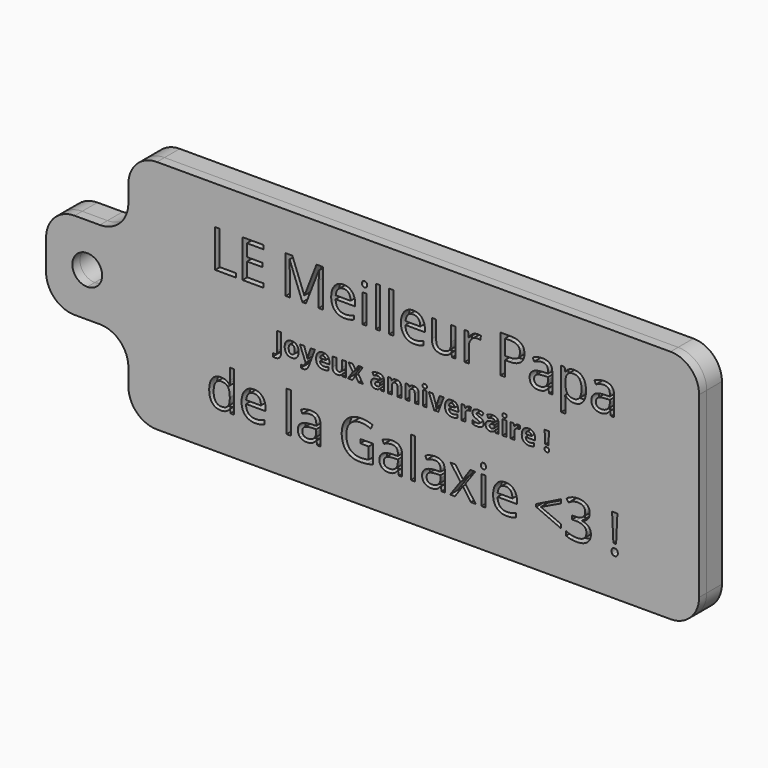
from build123d import *

# Parameters (mm, degrees)
F0_W         = 0.4505208333
F0_H         = 4.2213541667
F0_H_2       = 2.9730902778
F0_W_2       = 8.6528608203
F0_H_3       = 9.189594537
F1_DEPTH     = 1
F2_W         = 8.6528608203
F2_H         = 9.189594537
F3_DEPTH     = 2
F4_R         = 3
F4_2_R       = 3
F6_DEPTH     = 3.001
F7_TEXT_SIZE = 2.7777777778
F8_DEPTH     = 1


# Not quite as in the source:
# - Text() gives the source's letters only with a copy of the font that has no kerning and outlines rounded to 1/6400 em; it was checked with that copy


with BuildPart() as f1:
    # F0 (on Front) → F1 (new body)
    with BuildSketch(Plane.XZ):
        Polygon((-30, -12.3789965568), (30, -12.3789965568), (30, 12.3789965568), (-30, 12.3789965568), (-30, 4.5947972685), (-30, -4.5947972685), align=None)
        with BuildLine():
            Line((-19.2547743056, -8.3789965568), (-19.3146701389, -7.9805590568))
            Line((-19.3146701389, -7.9805590568), (-19.3389756944, -7.9805590568))
            add(Edge.make_bspline(
                [(-19.3389756944, -7.9805590568), (-19.6506076389, -8.4336840568), (-20.2721354167, -8.4336840568)],
                knots=[0, 0, 0, 1, 1, 1], degree=2))
            add(Edge.make_bspline(
                [(-20.2721354167, -8.4336840568), (-20.85546875, -8.4336840568), (-21.1796875, -8.034812529)],
                knots=[0, 0, 0, 1, 1, 1], degree=2))
            add(Edge.make_bspline(
                [(-21.1796875, -8.034812529), (-21.50390625, -7.6359410012), (-21.50390625, -6.9006979457)],
                knots=[0, 0, 0, 1, 1, 1], degree=2))
            add(Edge.make_bspline(
                [(-21.50390625, -6.9006979457), (-21.50390625, -6.1654548901), (-21.1783854167, -5.7583368345)],
                knots=[0, 0, 0, 1, 1, 1], degree=2))
            add(Edge.make_bspline(
                [(-21.1783854167, -5.7583368345), (-20.8528645833, -5.351218779), (-20.2721354167, -5.351218779)],
                knots=[0, 0, 0, 1, 1, 1], degree=2))
            add(Edge.make_bspline(
                [(-20.2721354167, -5.351218779), (-19.6671006944, -5.351218779), (-19.3441840278, -5.7913229457)],
                knots=[0, 0, 0, 1, 1, 1], degree=2))
            Line((-19.3441840278, -5.7913229457), (-19.30859375, -5.7913229457))
            Line((-19.30859375, -5.7913229457), (-19.3276909722, -5.5769132234))
            Line((-19.3276909722, -5.5769132234), (-19.3389756944, -5.3677118345))
            Line((-19.3389756944, -5.3677118345), (-19.3389756944, -4.1576423901))
            Line((-19.3389756944, -4.1576423901), (-18.8884548611, -4.1576423901))
            Line((-18.8884548611, -4.1576423901), (-18.8884548611, -8.3789965568))
            Line((-18.8884548611, -8.3789965568), (-19.2547743056, -8.3789965568))
        make_face(mode=Mode.SUBTRACT)
        with BuildLine():
            add(Edge.make_bspline(
                [(-16.1636284722, -8.3885451679), (-16.3763020833, -8.4336840568), (-16.6775173611, -8.4336840568)],
                knots=[0, 0, 0, 1, 1, 1], degree=2))
            add(Edge.make_bspline(
                [(-16.6775173611, -8.4336840568), (-17.3363715278, -8.4336840568), (-17.7178819444, -8.0317743345)],
                knots=[0, 0, 0, 1, 1, 1], degree=2))
            add(Edge.make_bspline(
                [(-17.7178819444, -8.0317743345), (-18.0993923611, -7.6298646123), (-18.0993923611, -6.9171910012)],
                knots=[0, 0, 0, 1, 1, 1], degree=2))
            add(Edge.make_bspline(
                [(-18.0993923611, -6.9171910012), (-18.0993923611, -6.1975729457), (-17.7452256944, -5.7743958623)],
                knots=[0, 0, 0, 1, 1, 1], degree=2))
            add(Edge.make_bspline(
                [(-17.7452256944, -5.7743958623), (-17.3910590278, -5.351218779), (-16.7938368056, -5.351218779)],
                knots=[0, 0, 0, 1, 1, 1], degree=2))
            add(Edge.make_bspline(
                [(-16.7938368056, -5.351218779), (-16.2356770833, -5.351218779), (-15.91015625, -5.7188403068)],
                knots=[0, 0, 0, 1, 1, 1], degree=2))
            add(Edge.make_bspline(
                [(-15.91015625, -5.7188403068), (-15.5846354167, -6.0864618345), (-15.5846354167, -6.6888923901)],
                knots=[0, 0, 0, 1, 1, 1], degree=2))
            Line((-15.5846354167, -6.6888923901), (-15.5846354167, -6.9736146123))
            Line((-15.5846354167, -6.9736146123), (-17.6323784722, -6.9736146123))
            add(Edge.make_bspline(
                [(-17.6323784722, -6.9736146123), (-17.6184895833, -7.4970521123), (-17.3676215278, -7.7683194734)],
                knots=[0, 0, 0, 1, 1, 1], degree=2))
            add(Edge.make_bspline(
                [(-17.3676215278, -7.7683194734), (-17.1167534722, -8.0395868345), (-16.6610243056, -8.0395868345)],
                knots=[0, 0, 0, 1, 1, 1], degree=2))
            add(Edge.make_bspline(
                [(-16.6610243056, -8.0395868345), (-16.1809895833, -8.0395868345), (-15.7122395833, -7.8390660012)],
                knots=[0, 0, 0, 1, 1, 1], degree=2))
            Line((-15.7122395833, -7.8390660012), (-15.7122395833, -8.2409757234))
            add(Edge.make_bspline(
                [(-15.7122395833, -8.2409757234), (-15.9509548611, -8.343406279), (-16.1636284722, -8.3885451679)],
                knots=[0, 0, 0, 1, 1, 1], degree=2))
        make_face(mode=Mode.SUBTRACT)
        with Locations((-13.1475694444, -6.2683194734)):
            Rectangle(F0_W, F0_H, mode=Mode.SUBTRACT)
        with BuildLine():
            Line((-9.8051215278, -8.3789965568), (-10.1393229167, -8.3789965568))
            Line((-10.1393229167, -8.3789965568), (-10.2287326389, -7.9553854457))
            Line((-10.2287326389, -7.9553854457), (-10.2504340278, -7.9553854457))
            add(Edge.make_bspline(
                [(-10.2504340278, -7.9553854457), (-10.47265625, -8.2348993345), (-10.6935763889, -8.3342916957)],
                knots=[0, 0, 0, 1, 1, 1], degree=2))
            add(Edge.make_bspline(
                [(-10.6935763889, -8.3342916957), (-10.9144965278, -8.4336840568), (-11.24609375, -8.4336840568)],
                knots=[0, 0, 0, 1, 1, 1], degree=2))
            add(Edge.make_bspline(
                [(-11.24609375, -8.4336840568), (-11.6879340278, -8.4336840568), (-11.9388020833, -8.2053854457)],
                knots=[0, 0, 0, 1, 1, 1], degree=2))
            add(Edge.make_bspline(
                [(-11.9388020833, -8.2053854457), (-12.1896701389, -7.9770868345), (-12.1896701389, -7.5569479457)],
                knots=[0, 0, 0, 1, 1, 1], degree=2))
            add(Edge.make_bspline(
                [(-12.1896701389, -7.5569479457), (-12.1896701389, -6.6567743345), (-10.7495659722, -6.6133715568)],
                knots=[0, 0, 0, 1, 1, 1], degree=2))
            Line((-10.7495659722, -6.6133715568), (-10.2452256944, -6.5968785012))
            Line((-10.2452256944, -6.5968785012), (-10.2452256944, -6.4119826679))
            add(Edge.make_bspline(
                [(-10.2452256944, -6.4119826679), (-10.2452256944, -6.062156279), (-10.3953993056, -5.8954896123)],
                knots=[0, 0, 0, 1, 1, 1], degree=2))
            add(Edge.make_bspline(
                [(-10.3953993056, -5.8954896123), (-10.5455729167, -5.7288229457), (-10.8771701389, -5.7288229457)],
                knots=[0, 0, 0, 1, 1, 1], degree=2))
            add(Edge.make_bspline(
                [(-10.8771701389, -5.7288229457), (-11.2486979167, -5.7288229457), (-11.7174479167, -5.9562535012)],
                knots=[0, 0, 0, 1, 1, 1], degree=2))
            Line((-11.7174479167, -5.9562535012), (-11.8563368056, -5.6116354457))
            add(Edge.make_bspline(
                [(-11.8563368056, -5.6116354457), (-11.63671875, -5.4927118345), (-11.375, -5.4250035012)],
                knots=[0, 0, 0, 1, 1, 1], degree=2))
            add(Edge.make_bspline(
                [(-11.375, -5.4250035012), (-11.11328125, -5.3572951679), (-10.8493923611, -5.3572951679)],
                knots=[0, 0, 0, 1, 1, 1], degree=2))
            add(Edge.make_bspline(
                [(-10.8493923611, -5.3572951679), (-10.3181423611, -5.3572951679), (-10.0616319444, -5.5929722512)],
                knots=[0, 0, 0, 1, 1, 1], degree=2))
            add(Edge.make_bspline(
                [(-10.0616319444, -5.5929722512), (-9.8051215278, -5.8286493345), (-9.8051215278, -6.3494826679)],
                knots=[0, 0, 0, 1, 1, 1], degree=2))
            Line((-9.8051215278, -6.3494826679), (-9.8051215278, -8.3789965568))
        make_face(mode=Mode.SUBTRACT)
        with BuildLine():
            Line((-5.6219618056, -6.7131979457), (-5.6219618056, -6.3008715568))
            Line((-5.6219618056, -6.3008715568), (-4.2738715278, -6.3008715568))
            Line((-4.2738715278, -6.3008715568), (-4.2738715278, -8.2296910012))
            add(Edge.make_bspline(
                [(-4.2738715278, -8.2296910012), (-4.5889756944, -8.3303854457), (-4.9144965278, -8.3820347512)],
                knots=[0, 0, 0, 1, 1, 1], degree=2))
            add(Edge.make_bspline(
                [(-4.9144965278, -8.3820347512), (-5.2400173611, -8.4336840568), (-5.6688368056, -8.4336840568)],
                knots=[0, 0, 0, 1, 1, 1], degree=2))
            add(Edge.make_bspline(
                [(-5.6688368056, -8.4336840568), (-6.5690104167, -8.4336840568), (-7.0707465278, -7.8976597512)],
                knots=[0, 0, 0, 1, 1, 1], degree=2))
            add(Edge.make_bspline(
                [(-7.0707465278, -7.8976597512), (-7.5724826389, -7.3616354457), (-7.5724826389, -6.3963576679)],
                knots=[0, 0, 0, 1, 1, 1], degree=2))
            add(Edge.make_bspline(
                [(-7.5724826389, -6.3963576679), (-7.5724826389, -5.7774340568), (-7.32421875, -5.312156279)],
                knots=[0, 0, 0, 1, 1, 1], degree=2))
            add(Edge.make_bspline(
                [(-7.32421875, -5.312156279), (-7.0759548611, -4.8468785012), (-6.609375, -4.6016528068)],
                knots=[0, 0, 0, 1, 1, 1], degree=2))
            add(Edge.make_bspline(
                [(-6.609375, -4.6016528068), (-6.1427951389, -4.3564271123), (-5.5169270833, -4.3564271123)],
                knots=[0, 0, 0, 1, 1, 1], degree=2))
            add(Edge.make_bspline(
                [(-5.5169270833, -4.3564271123), (-4.8815104167, -4.3564271123), (-4.3337673611, -4.5890660012)],
                knots=[0, 0, 0, 1, 1, 1], degree=2))
            Line((-4.3337673611, -4.5890660012), (-4.5125868056, -4.9961840568))
            add(Edge.make_bspline(
                [(-4.5125868056, -4.9961840568), (-5.0499131944, -4.7687535012), (-5.5464409722, -4.7687535012)],
                knots=[0, 0, 0, 1, 1, 1], degree=2))
            add(Edge.make_bspline(
                [(-5.5464409722, -4.7687535012), (-6.2703993056, -4.7687535012), (-6.6775173611, -5.1997430845)],
                knots=[0, 0, 0, 1, 1, 1], degree=2))
            add(Edge.make_bspline(
                [(-6.6775173611, -5.1997430845), (-7.0846354167, -5.6307326679), (-7.0846354167, -6.3963576679)],
                knots=[0, 0, 0, 1, 1, 1], degree=2))
            add(Edge.make_bspline(
                [(-7.0846354167, -6.3963576679), (-7.0846354167, -7.1993090568), (-6.6927083333, -7.6142396123)],
                knots=[0, 0, 0, 1, 1, 1], degree=2))
            add(Edge.make_bspline(
                [(-6.6927083333, -7.6142396123), (-6.30078125, -8.0291701679), (-5.5412326389, -8.0291701679)],
                knots=[0, 0, 0, 1, 1, 1], degree=2))
            add(Edge.make_bspline(
                [(-5.5412326389, -8.0291701679), (-5.12890625, -8.0291701679), (-4.7356770833, -7.9336840568)],
                knots=[0, 0, 0, 1, 1, 1], degree=2))
            Line((-4.7356770833, -7.9336840568), (-4.7356770833, -6.7131979457))
            Line((-4.7356770833, -6.7131979457), (-5.6219618056, -6.7131979457))
        make_face(mode=Mode.SUBTRACT)
        with BuildLine():
            Line((-1.2278645833, -8.3789965568), (-1.5620659722, -8.3789965568))
            Line((-1.5620659722, -8.3789965568), (-1.6514756944, -7.9553854457))
            Line((-1.6514756944, -7.9553854457), (-1.6731770833, -7.9553854457))
            add(Edge.make_bspline(
                [(-1.6731770833, -7.9553854457), (-1.8953993056, -8.2348993345), (-2.1163194444, -8.3342916957)],
                knots=[0, 0, 0, 1, 1, 1], degree=2))
            add(Edge.make_bspline(
                [(-2.1163194444, -8.3342916957), (-2.3372395833, -8.4336840568), (-2.6688368056, -8.4336840568)],
                knots=[0, 0, 0, 1, 1, 1], degree=2))
            add(Edge.make_bspline(
                [(-2.6688368056, -8.4336840568), (-3.1106770833, -8.4336840568), (-3.3615451389, -8.2053854457)],
                knots=[0, 0, 0, 1, 1, 1], degree=2))
            add(Edge.make_bspline(
                [(-3.3615451389, -8.2053854457), (-3.6124131944, -7.9770868345), (-3.6124131944, -7.5569479457)],
                knots=[0, 0, 0, 1, 1, 1], degree=2))
            add(Edge.make_bspline(
                [(-3.6124131944, -7.5569479457), (-3.6124131944, -6.6567743345), (-2.1723090278, -6.6133715568)],
                knots=[0, 0, 0, 1, 1, 1], degree=2))
            Line((-2.1723090278, -6.6133715568), (-1.66796875, -6.5968785012))
            Line((-1.66796875, -6.5968785012), (-1.66796875, -6.4119826679))
            add(Edge.make_bspline(
                [(-1.66796875, -6.4119826679), (-1.66796875, -6.062156279), (-1.8181423611, -5.8954896123)],
                knots=[0, 0, 0, 1, 1, 1], degree=2))
            add(Edge.make_bspline(
                [(-1.8181423611, -5.8954896123), (-1.9683159722, -5.7288229457), (-2.2999131944, -5.7288229457)],
                knots=[0, 0, 0, 1, 1, 1], degree=2))
            add(Edge.make_bspline(
                [(-2.2999131944, -5.7288229457), (-2.6714409722, -5.7288229457), (-3.1401909722, -5.9562535012)],
                knots=[0, 0, 0, 1, 1, 1], degree=2))
            Line((-3.1401909722, -5.9562535012), (-3.2790798611, -5.6116354457))
            add(Edge.make_bspline(
                [(-3.2790798611, -5.6116354457), (-3.0594618056, -5.4927118345), (-2.7977430556, -5.4250035012)],
                knots=[0, 0, 0, 1, 1, 1], degree=2))
            add(Edge.make_bspline(
                [(-2.7977430556, -5.4250035012), (-2.5360243056, -5.3572951679), (-2.2721354167, -5.3572951679)],
                knots=[0, 0, 0, 1, 1, 1], degree=2))
            add(Edge.make_bspline(
                [(-2.2721354167, -5.3572951679), (-1.7408854167, -5.3572951679), (-1.484375, -5.5929722512)],
                knots=[0, 0, 0, 1, 1, 1], degree=2))
            add(Edge.make_bspline(
                [(-1.484375, -5.5929722512), (-1.2278645833, -5.8286493345), (-1.2278645833, -6.3494826679)],
                knots=[0, 0, 0, 1, 1, 1], degree=2))
            Line((-1.2278645833, -6.3494826679), (-1.2278645833, -8.3789965568))
        make_face(mode=Mode.SUBTRACT)
        with Locations((-0.0755208333, -6.2683194734)):
            Rectangle(F0_W, F0_H, mode=Mode.SUBTRACT)
        with BuildLine():
            Line((3.2669270833, -8.3789965568), (2.9327256944, -8.3789965568))
            Line((2.9327256944, -8.3789965568), (2.8433159722, -7.9553854457))
            Line((2.8433159722, -7.9553854457), (2.8216145833, -7.9553854457))
            add(Edge.make_bspline(
                [(2.8216145833, -7.9553854457), (2.5993923611, -8.2348993345), (2.3784722222, -8.3342916957)],
                knots=[0, 0, 0, 1, 1, 1], degree=2))
            add(Edge.make_bspline(
                [(2.3784722222, -8.3342916957), (2.1575520833, -8.4336840568), (1.8259548611, -8.4336840568)],
                knots=[0, 0, 0, 1, 1, 1], degree=2))
            add(Edge.make_bspline(
                [(1.8259548611, -8.4336840568), (1.3841145833, -8.4336840568), (1.1332465278, -8.2053854457)],
                knots=[0, 0, 0, 1, 1, 1], degree=2))
            add(Edge.make_bspline(
                [(1.1332465278, -8.2053854457), (0.8823784722, -7.9770868345), (0.8823784722, -7.5569479457)],
                knots=[0, 0, 0, 1, 1, 1], degree=2))
            add(Edge.make_bspline(
                [(0.8823784722, -7.5569479457), (0.8823784722, -6.6567743345), (2.3224826389, -6.6133715568)],
                knots=[0, 0, 0, 1, 1, 1], degree=2))
            Line((2.3224826389, -6.6133715568), (2.8268229167, -6.5968785012))
            Line((2.8268229167, -6.5968785012), (2.8268229167, -6.4119826679))
            add(Edge.make_bspline(
                [(2.8268229167, -6.4119826679), (2.8268229167, -6.062156279), (2.6766493056, -5.8954896123)],
                knots=[0, 0, 0, 1, 1, 1], degree=2))
            add(Edge.make_bspline(
                [(2.6766493056, -5.8954896123), (2.5264756944, -5.7288229457), (2.1948784722, -5.7288229457)],
                knots=[0, 0, 0, 1, 1, 1], degree=2))
            add(Edge.make_bspline(
                [(2.1948784722, -5.7288229457), (1.8233506944, -5.7288229457), (1.3546006944, -5.9562535012)],
                knots=[0, 0, 0, 1, 1, 1], degree=2))
            Line((1.3546006944, -5.9562535012), (1.2157118056, -5.6116354457))
            add(Edge.make_bspline(
                [(1.2157118056, -5.6116354457), (1.4353298611, -5.4927118345), (1.6970486111, -5.4250035012)],
                knots=[0, 0, 0, 1, 1, 1], degree=2))
            add(Edge.make_bspline(
                [(1.6970486111, -5.4250035012), (1.9587673611, -5.3572951679), (2.22265625, -5.3572951679)],
                knots=[0, 0, 0, 1, 1, 1], degree=2))
            add(Edge.make_bspline(
                [(2.22265625, -5.3572951679), (2.75390625, -5.3572951679), (3.0104166667, -5.5929722512)],
                knots=[0, 0, 0, 1, 1, 1], degree=2))
            add(Edge.make_bspline(
                [(3.0104166667, -5.5929722512), (3.2669270833, -5.8286493345), (3.2669270833, -6.3494826679)],
                knots=[0, 0, 0, 1, 1, 1], degree=2))
            Line((3.2669270833, -6.3494826679), (3.2669270833, -8.3789965568))
        make_face(mode=Mode.SUBTRACT)
        Polygon((3.8224826389, -8.3789965568), (4.91015625, -6.8572951679), (3.8763020833, -5.405906279), (4.3893229167, -5.405906279), (5.1731770833, -6.5447951679), (5.9544270833, -5.405906279), (6.4622395833, -5.405906279), (5.4283854167, -6.8572951679), (6.5160590278, -8.3789965568), (6.0065104167, -8.3789965568), (5.1731770833, -7.1741354457), (4.33203125, -8.3789965568), align=None, mode=Mode.SUBTRACT)
        with Locations((7.3298611111, -6.8924514179)):
            Rectangle(F0_W, F0_H_2, mode=Mode.SUBTRACT)
        with BuildLine():
            add(Edge.make_bspline(
                [(10.2799479167, -8.3885451679), (10.0672743056, -8.4336840568), (9.7660590278, -8.4336840568)],
                knots=[0, 0, 0, 1, 1, 1], degree=2))
            add(Edge.make_bspline(
                [(9.7660590278, -8.4336840568), (9.1072048611, -8.4336840568), (8.7256944444, -8.0317743345)],
                knots=[0, 0, 0, 1, 1, 1], degree=2))
            add(Edge.make_bspline(
                [(8.7256944444, -8.0317743345), (8.3441840278, -7.6298646123), (8.3441840278, -6.9171910012)],
                knots=[0, 0, 0, 1, 1, 1], degree=2))
            add(Edge.make_bspline(
                [(8.3441840278, -6.9171910012), (8.3441840278, -6.1975729457), (8.6983506944, -5.7743958623)],
                knots=[0, 0, 0, 1, 1, 1], degree=2))
            add(Edge.make_bspline(
                [(8.6983506944, -5.7743958623), (9.0525173611, -5.351218779), (9.6497395833, -5.351218779)],
                knots=[0, 0, 0, 1, 1, 1], degree=2))
            add(Edge.make_bspline(
                [(9.6497395833, -5.351218779), (10.2078993056, -5.351218779), (10.5334201389, -5.7188403068)],
                knots=[0, 0, 0, 1, 1, 1], degree=2))
            add(Edge.make_bspline(
                [(10.5334201389, -5.7188403068), (10.8589409722, -6.0864618345), (10.8589409722, -6.6888923901)],
                knots=[0, 0, 0, 1, 1, 1], degree=2))
            Line((10.8589409722, -6.6888923901), (10.8589409722, -6.9736146123))
            Line((10.8589409722, -6.9736146123), (8.8111979167, -6.9736146123))
            add(Edge.make_bspline(
                [(8.8111979167, -6.9736146123), (8.8250868056, -7.4970521123), (9.0759548611, -7.7683194734)],
                knots=[0, 0, 0, 1, 1, 1], degree=2))
            add(Edge.make_bspline(
                [(9.0759548611, -7.7683194734), (9.3268229167, -8.0395868345), (9.7825520833, -8.0395868345)],
                knots=[0, 0, 0, 1, 1, 1], degree=2))
            add(Edge.make_bspline(
                [(9.7825520833, -8.0395868345), (10.2625868056, -8.0395868345), (10.7313368056, -7.8390660012)],
                knots=[0, 0, 0, 1, 1, 1], degree=2))
            Line((10.7313368056, -7.8390660012), (10.7313368056, -8.2409757234))
            add(Edge.make_bspline(
                [(10.7313368056, -8.2409757234), (10.4926215278, -8.343406279), (10.2799479167, -8.3885451679)],
                knots=[0, 0, 0, 1, 1, 1], degree=2))
        make_face(mode=Mode.SUBTRACT)
        with BuildLine():
            add(Edge.make_bspline(
                [(20.8940972222, -8.3724861401), (20.8016493056, -8.2869826679), (20.8016493056, -8.0916701679)],
                knots=[0, 0, 0, 1, 1, 1], degree=2))
            add(Edge.make_bspline(
                [(20.8016493056, -8.0916701679), (20.8016493056, -7.7227465568), (21.1271701389, -7.7227465568)],
                knots=[0, 0, 0, 1, 1, 1], degree=2))
            add(Edge.make_bspline(
                [(21.1271701389, -7.7227465568), (21.2842881944, -7.7227465568), (21.3697916667, -7.8173646123)],
                knots=[0, 0, 0, 1, 1, 1], degree=2))
            add(Edge.make_bspline(
                [(21.3697916667, -7.8173646123), (21.4552951389, -7.9119826679), (21.4552951389, -8.0916701679)],
                knots=[0, 0, 0, 1, 1, 1], degree=2))
            add(Edge.make_bspline(
                [(21.4552951389, -8.0916701679), (21.4552951389, -8.265281279), (21.3684895833, -8.3616354457)],
                knots=[0, 0, 0, 1, 1, 1], degree=2))
            add(Edge.make_bspline(
                [(21.3684895833, -8.3616354457), (21.2816840278, -8.4579896123), (21.1271701389, -8.4579896123)],
                knots=[0, 0, 0, 1, 1, 1], degree=2))
            add(Edge.make_bspline(
                [(21.1271701389, -8.4579896123), (20.9865451389, -8.4579896123), (20.8940972222, -8.3724861401)],
                knots=[0, 0, 0, 1, 1, 1], degree=2))
        make_face(mode=Mode.SUBTRACT)
        Polygon((15.4822048611, -7.3130243345), (15.4822048611, -7.7227465568), (12.8754340278, -6.577781279), (12.8754340278, -6.312156279), (15.4822048611, -5.0126771123), (15.4822048611, -5.4163229457), (13.3606770833, -6.4232673901), align=None, mode=Mode.SUBTRACT)
        with BuildLine():
            add(Edge.make_bspline(
                [(18.1783854167, -4.620750029), (18.4986979167, -4.8850729457), (18.4986979167, -5.3460104457)],
                knots=[0, 0, 0, 1, 1, 1], degree=2))
            add(Edge.make_bspline(
                [(18.4986979167, -5.3460104457), (18.4986979167, -5.726218779), (18.2855902778, -5.9675382234)],
                knots=[0, 0, 0, 1, 1, 1], degree=2))
            add(Edge.make_bspline(
                [(18.2855902778, -5.9675382234), (18.0724826389, -6.2088576679), (17.6818576389, -6.2904548901)],
                knots=[0, 0, 0, 1, 1, 1], degree=2))
            Line((17.6818576389, -6.2904548901), (17.6818576389, -6.312156279))
            add(Edge.make_bspline(
                [(17.6818576389, -6.312156279), (18.1592881944, -6.3711840568), (18.3897569444, -6.6155416957)],
                knots=[0, 0, 0, 1, 1, 1], degree=2))
            add(Edge.make_bspline(
                [(18.3897569444, -6.6155416957), (18.6202256944, -6.8598993345), (18.6202256944, -7.2557326679)],
                knots=[0, 0, 0, 1, 1, 1], degree=2))
            add(Edge.make_bspline(
                [(18.6202256944, -7.2557326679), (18.6202256944, -7.8225729457), (18.2269965278, -8.1281285012)],
                knots=[0, 0, 0, 1, 1, 1], degree=2))
            add(Edge.make_bspline(
                [(18.2269965278, -8.1281285012), (17.8337673611, -8.4336840568), (17.1098090278, -8.4336840568)],
                knots=[0, 0, 0, 1, 1, 1], degree=2))
            add(Edge.make_bspline(
                [(17.1098090278, -8.4336840568), (16.7947048611, -8.4336840568), (16.5329861111, -8.3859410012)],
                knots=[0, 0, 0, 1, 1, 1], degree=2))
            add(Edge.make_bspline(
                [(16.5329861111, -8.3859410012), (16.2712673611, -8.3381979457), (16.0247395833, -8.2192743345)],
                knots=[0, 0, 0, 1, 1, 1], degree=2))
            Line((16.0247395833, -8.2192743345), (16.0247395833, -7.7904548901))
            add(Edge.make_bspline(
                [(16.0247395833, -7.7904548901), (16.2825520833, -7.9180590568), (16.57421875, -7.9844653068)],
                knots=[0, 0, 0, 1, 1, 1], degree=2))
            add(Edge.make_bspline(
                [(16.57421875, -7.9844653068), (16.8658854167, -8.0508715568), (17.1263020833, -8.0508715568)],
                knots=[0, 0, 0, 1, 1, 1], degree=2))
            add(Edge.make_bspline(
                [(17.1263020833, -8.0508715568), (18.1540798611, -8.0508715568), (18.1540798611, -7.2453160012)],
                knots=[0, 0, 0, 1, 1, 1], degree=2))
            add(Edge.make_bspline(
                [(18.1540798611, -7.2453160012), (18.1540798611, -6.523093779), (17.0203993056, -6.523093779)],
                knots=[0, 0, 0, 1, 1, 1], degree=2))
            Line((17.0203993056, -6.523093779), (16.6297743056, -6.523093779))
            Line((16.6297743056, -6.523093779), (16.6297743056, -6.1359410012))
            Line((16.6297743056, -6.1359410012), (17.0256076389, -6.1359410012))
            add(Edge.make_bspline(
                [(17.0256076389, -6.1359410012), (17.4891493056, -6.1359410012), (17.7604166667, -5.9310798901)],
                knots=[0, 0, 0, 1, 1, 1], degree=2))
            add(Edge.make_bspline(
                [(17.7604166667, -5.9310798901), (18.0316840278, -5.726218779), (18.0316840278, -5.3625035012)],
                knots=[0, 0, 0, 1, 1, 1], degree=2))
            add(Edge.make_bspline(
                [(18.0316840278, -5.3625035012), (18.0316840278, -5.0725729457), (17.8324652778, -4.9067743345)],
                knots=[0, 0, 0, 1, 1, 1], degree=2))
            add(Edge.make_bspline(
                [(17.8324652778, -4.9067743345), (17.6332465278, -4.7409757234), (17.2912326389, -4.7409757234)],
                knots=[0, 0, 0, 1, 1, 1], degree=2))
            add(Edge.make_bspline(
                [(17.2912326389, -4.7409757234), (17.0308159722, -4.7409757234), (16.8003472222, -4.8117222512)],
                knots=[0, 0, 0, 1, 1, 1], degree=2))
            add(Edge.make_bspline(
                [(16.8003472222, -4.8117222512), (16.5698784722, -4.882468779), (16.2738715278, -5.0725729457)],
                knots=[0, 0, 0, 1, 1, 1], degree=2))
            Line((16.2738715278, -5.0725729457), (16.0464409722, -4.7687535012))
            add(Edge.make_bspline(
                [(16.0464409722, -4.7687535012), (16.2903645833, -4.5760451679), (16.6089409722, -4.4662361401)],
                knots=[0, 0, 0, 1, 1, 1], degree=2))
            add(Edge.make_bspline(
                [(16.6089409722, -4.4662361401), (16.9275173611, -4.3564271123), (17.2808159722, -4.3564271123)],
                knots=[0, 0, 0, 1, 1, 1], degree=2))
            add(Edge.make_bspline(
                [(17.2808159722, -4.3564271123), (17.8580729167, -4.3564271123), (18.1783854167, -4.620750029)],
                knots=[0, 0, 0, 1, 1, 1], degree=2))
        make_face(mode=Mode.SUBTRACT)
        with BuildLine():
            add(Edge.make_bspline(
                [(7.1423611111, -4.8269132234), (7.06640625, -4.7522604457), (7.06640625, -4.6003507234)],
                knots=[0, 0, 0, 1, 1, 1], degree=2))
            add(Edge.make_bspline(
                [(7.06640625, -4.6003507234), (7.06640625, -4.4458368345), (7.1423611111, -4.3737882234)],
                knots=[0, 0, 0, 1, 1, 1], degree=2))
            add(Edge.make_bspline(
                [(7.1423611111, -4.3737882234), (7.2183159722, -4.3017396123), (7.3328993056, -4.3017396123)],
                knots=[0, 0, 0, 1, 1, 1], degree=2))
            add(Edge.make_bspline(
                [(7.3328993056, -4.3017396123), (7.44140625, -4.3017396123), (7.5199652778, -4.3750903068)],
                knots=[0, 0, 0, 1, 1, 1], degree=2))
            add(Edge.make_bspline(
                [(7.5199652778, -4.3750903068), (7.5985243056, -4.4484410012), (7.5985243056, -4.6003507234)],
                knots=[0, 0, 0, 1, 1, 1], degree=2))
            add(Edge.make_bspline(
                [(7.5985243056, -4.6003507234), (7.5985243056, -4.7522604457), (7.5199652778, -4.8269132234)],
                knots=[0, 0, 0, 1, 1, 1], degree=2))
            add(Edge.make_bspline(
                [(7.5199652778, -4.8269132234), (7.44140625, -4.9015660012), (7.3328993056, -4.9015660012)],
                knots=[0, 0, 0, 1, 1, 1], degree=2))
            add(Edge.make_bspline(
                [(7.3328993056, -4.9015660012), (7.2183159722, -4.9015660012), (7.1423611111, -4.8269132234)],
                knots=[0, 0, 0, 1, 1, 1], degree=2))
        make_face(mode=Mode.SUBTRACT)
        Polygon((21.4118923611, -4.4128507234), (21.2738715278, -7.2861146123), (20.9891493056, -7.2861146123), (20.8502604167, -4.4128507234), align=None, mode=Mode.SUBTRACT)
        with BuildLine():
            add(Edge.make_bspline(
                [(-6.7417534722, 4.3694479457), (-6.9544270833, 4.3243090568), (-7.2556423611, 4.3243090568)],
                knots=[0, 0, 0, 1, 1, 1], degree=2))
            add(Edge.make_bspline(
                [(-7.2556423611, 4.3243090568), (-7.9144965278, 4.3243090568), (-8.2960069444, 4.726218779)],
                knots=[0, 0, 0, 1, 1, 1], degree=2))
            add(Edge.make_bspline(
                [(-8.2960069444, 4.726218779), (-8.6775173611, 5.1281285012), (-8.6775173611, 5.8408021123)],
                knots=[0, 0, 0, 1, 1, 1], degree=2))
            add(Edge.make_bspline(
                [(-8.6775173611, 5.8408021123), (-8.6775173611, 6.5604201679), (-8.3233506944, 6.9835972512)],
                knots=[0, 0, 0, 1, 1, 1], degree=2))
            add(Edge.make_bspline(
                [(-8.3233506944, 6.9835972512), (-7.9691840278, 7.4067743345), (-7.3719618056, 7.4067743345)],
                knots=[0, 0, 0, 1, 1, 1], degree=2))
            add(Edge.make_bspline(
                [(-7.3719618056, 7.4067743345), (-6.8138020833, 7.4067743345), (-6.48828125, 7.0391528068)],
                knots=[0, 0, 0, 1, 1, 1], degree=2))
            add(Edge.make_bspline(
                [(-6.48828125, 7.0391528068), (-6.1627604167, 6.671531279), (-6.1627604167, 6.0691007234)],
                knots=[0, 0, 0, 1, 1, 1], degree=2))
            Line((-6.1627604167, 6.0691007234), (-6.1627604167, 5.7843785012))
            Line((-6.1627604167, 5.7843785012), (-8.2105034722, 5.7843785012))
            add(Edge.make_bspline(
                [(-8.2105034722, 5.7843785012), (-8.1966145833, 5.2609410012), (-7.9457465278, 4.9896736401)],
                knots=[0, 0, 0, 1, 1, 1], degree=2))
            add(Edge.make_bspline(
                [(-7.9457465278, 4.9896736401), (-7.6948784722, 4.718406279), (-7.2391493056, 4.718406279)],
                knots=[0, 0, 0, 1, 1, 1], degree=2))
            add(Edge.make_bspline(
                [(-7.2391493056, 4.718406279), (-6.7591145833, 4.718406279), (-6.2903645833, 4.9189271123)],
                knots=[0, 0, 0, 1, 1, 1], degree=2))
            Line((-6.2903645833, 4.9189271123), (-6.2903645833, 4.5170173901))
            add(Edge.make_bspline(
                [(-6.2903645833, 4.5170173901), (-6.5290798611, 4.4145868345), (-6.7417534722, 4.3694479457)],
                knots=[0, 0, 0, 1, 1, 1], degree=2))
        make_face(mode=Mode.SUBTRACT)
        with Locations((-5.1692708333, 5.8655416957)):
            Rectangle(F0_W, F0_H_2, mode=Mode.SUBTRACT)
        Polygon((-18.6653645833, 4.3789965568), (-20.8763020833, 4.3789965568), (-20.8763020833, 8.3451423901), (-20.4153645833, 8.3451423901), (-20.4153645833, 4.796531279), (-18.6653645833, 4.796531279), align=None, mode=Mode.SUBTRACT)
        Polygon((-15.7816840278, 4.7913229457), (-15.7816840278, 4.3789965568), (-17.9926215278, 4.3789965568), (-17.9926215278, 8.3451423901), (-15.7816840278, 8.3451423901), (-15.7816840278, 7.9354201679), (-17.5316840278, 7.9354201679), (-17.5316840278, 6.6576423901), (-15.8875868056, 6.6576423901), (-15.8875868056, 6.2505243345), (-17.5316840278, 6.2505243345), (-17.5316840278, 4.7913229457), align=None, mode=Mode.SUBTRACT)
        with BuildLine():
            Line((-11.3328993056, 4.3789965568), (-11.7044270833, 4.3789965568))
            Line((-11.7044270833, 4.3789965568), (-13.0499131944, 7.8946215568))
            Line((-13.0499131944, 7.8946215568), (-13.0716145833, 7.8946215568))
            add(Edge.make_bspline(
                [(-13.0716145833, 7.8946215568), (-13.0334201389, 7.4770868345), (-13.0334201389, 6.9015660012)],
                knots=[0, 0, 0, 1, 1, 1], degree=2))
            Line((-13.0334201389, 6.9015660012), (-13.0334201389, 4.3789965568))
            Line((-13.0334201389, 4.3789965568), (-13.4596354167, 4.3789965568))
            Line((-13.4596354167, 4.3789965568), (-13.4596354167, 8.3451423901))
            Line((-13.4596354167, 8.3451423901), (-12.7651909722, 8.3451423901))
            Line((-12.7651909722, 8.3451423901), (-11.5091145833, 5.0734410012))
            Line((-11.5091145833, 5.0734410012), (-11.4874131944, 5.0734410012))
            Line((-11.4874131944, 5.0734410012), (-10.2209201389, 8.3451423901))
            Line((-10.2209201389, 8.3451423901), (-9.5316840278, 8.3451423901))
            Line((-9.5316840278, 8.3451423901), (-9.5316840278, 4.3789965568))
            Line((-9.5316840278, 4.3789965568), (-9.9926215278, 4.3789965568))
            Line((-9.9926215278, 4.3789965568), (-9.9926215278, 6.9345521123))
            add(Edge.make_bspline(
                [(-9.9926215278, 6.9345521123), (-9.9926215278, 7.3737882234), (-9.9544270833, 7.8894132234)],
                knots=[0, 0, 0, 1, 1, 1], degree=2))
            Line((-9.9544270833, 7.8894132234), (-9.9761284722, 7.8894132234))
            Line((-9.9761284722, 7.8894132234), (-11.3328993056, 4.3789965568))
        make_face(mode=Mode.SUBTRACT)
        with BuildLine():
            add(Edge.make_bspline(
                [(-5.3567708333, 7.9310798901), (-5.4327256944, 8.0057326679), (-5.4327256944, 8.1576423901)],
                knots=[0, 0, 0, 1, 1, 1], degree=2))
            add(Edge.make_bspline(
                [(-5.4327256944, 8.1576423901), (-5.4327256944, 8.312156279), (-5.3567708333, 8.3842048901)],
                knots=[0, 0, 0, 1, 1, 1], degree=2))
            add(Edge.make_bspline(
                [(-5.3567708333, 8.3842048901), (-5.2808159722, 8.4562535012), (-5.1662326389, 8.4562535012)],
                knots=[0, 0, 0, 1, 1, 1], degree=2))
            add(Edge.make_bspline(
                [(-5.1662326389, 8.4562535012), (-5.0577256944, 8.4562535012), (-4.9791666667, 8.3829028068)],
                knots=[0, 0, 0, 1, 1, 1], degree=2))
            add(Edge.make_bspline(
                [(-4.9791666667, 8.3829028068), (-4.9006076389, 8.3095521123), (-4.9006076389, 8.1576423901)],
                knots=[0, 0, 0, 1, 1, 1], degree=2))
            add(Edge.make_bspline(
                [(-4.9006076389, 8.1576423901), (-4.9006076389, 8.0057326679), (-4.9791666667, 7.9310798901)],
                knots=[0, 0, 0, 1, 1, 1], degree=2))
            add(Edge.make_bspline(
                [(-4.9791666667, 7.9310798901), (-5.0577256944, 7.8564271123), (-5.1662326389, 7.8564271123)],
                knots=[0, 0, 0, 1, 1, 1], degree=2))
            add(Edge.make_bspline(
                [(-5.1662326389, 7.8564271123), (-5.2808159722, 7.8564271123), (-5.3567708333, 7.9310798901)],
                knots=[0, 0, 0, 1, 1, 1], degree=2))
        make_face(mode=Mode.SUBTRACT)
        with BuildLine():
            add(Edge.make_bspline(
                [(0.5915798611, 4.3694479457), (0.37890625, 4.3243090568), (0.0776909722, 4.3243090568)],
                knots=[0, 0, 0, 1, 1, 1], degree=2))
            add(Edge.make_bspline(
                [(0.0776909722, 4.3243090568), (-0.5811631944, 4.3243090568), (-0.9626736111, 4.726218779)],
                knots=[0, 0, 0, 1, 1, 1], degree=2))
            add(Edge.make_bspline(
                [(-0.9626736111, 4.726218779), (-1.3441840278, 5.1281285012), (-1.3441840278, 5.8408021123)],
                knots=[0, 0, 0, 1, 1, 1], degree=2))
            add(Edge.make_bspline(
                [(-1.3441840278, 5.8408021123), (-1.3441840278, 6.5604201679), (-0.9900173611, 6.9835972512)],
                knots=[0, 0, 0, 1, 1, 1], degree=2))
            add(Edge.make_bspline(
                [(-0.9900173611, 6.9835972512), (-0.6358506944, 7.4067743345), (-0.0386284722, 7.4067743345)],
                knots=[0, 0, 0, 1, 1, 1], degree=2))
            add(Edge.make_bspline(
                [(-0.0386284722, 7.4067743345), (0.51953125, 7.4067743345), (0.8450520833, 7.0391528068)],
                knots=[0, 0, 0, 1, 1, 1], degree=2))
            add(Edge.make_bspline(
                [(0.8450520833, 7.0391528068), (1.1705729167, 6.671531279), (1.1705729167, 6.0691007234)],
                knots=[0, 0, 0, 1, 1, 1], degree=2))
            Line((1.1705729167, 6.0691007234), (1.1705729167, 5.7843785012))
            Line((1.1705729167, 5.7843785012), (-0.8771701389, 5.7843785012))
            add(Edge.make_bspline(
                [(-0.8771701389, 5.7843785012), (-0.86328125, 5.2609410012), (-0.6124131944, 4.9896736401)],
                knots=[0, 0, 0, 1, 1, 1], degree=2))
            add(Edge.make_bspline(
                [(-0.6124131944, 4.9896736401), (-0.3615451389, 4.718406279), (0.0941840278, 4.718406279)],
                knots=[0, 0, 0, 1, 1, 1], degree=2))
            add(Edge.make_bspline(
                [(0.0941840278, 4.718406279), (0.57421875, 4.718406279), (1.04296875, 4.9189271123)],
                knots=[0, 0, 0, 1, 1, 1], degree=2))
            Line((1.04296875, 4.9189271123), (1.04296875, 4.5170173901))
            add(Edge.make_bspline(
                [(1.04296875, 4.5170173901), (0.8042534722, 4.4145868345), (0.5915798611, 4.3694479457)],
                knots=[0, 0, 0, 1, 1, 1], degree=2))
        make_face(mode=Mode.SUBTRACT)
        with BuildLine():
            Line((1.9066840278, 7.3520868345), (2.3624131944, 7.3520868345))
            Line((2.3624131944, 7.3520868345), (2.3624131944, 5.4232673901))
            add(Edge.make_bspline(
                [(2.3624131944, 5.4232673901), (2.3624131944, 5.0595521123), (2.5277777778, 4.8807326679)],
                knots=[0, 0, 0, 1, 1, 1], degree=2))
            add(Edge.make_bspline(
                [(2.5277777778, 4.8807326679), (2.6931423611, 4.7019132234), (3.0455729167, 4.7019132234)],
                knots=[0, 0, 0, 1, 1, 1], degree=2))
            add(Edge.make_bspline(
                [(3.0455729167, 4.7019132234), (3.5125868056, 4.7019132234), (3.7278645833, 4.956687529)],
                knots=[0, 0, 0, 1, 1, 1], degree=2))
            add(Edge.make_bspline(
                [(3.7278645833, 4.956687529), (3.9431423611, 5.2114618345), (3.9431423611, 5.7895868345)],
                knots=[0, 0, 0, 1, 1, 1], degree=2))
            Line((3.9431423611, 5.7895868345), (3.9431423611, 7.3520868345))
            Line((3.9431423611, 7.3520868345), (4.3936631944, 7.3520868345))
            Line((4.3936631944, 7.3520868345), (4.3936631944, 4.3789965568))
            Line((4.3936631944, 4.3789965568), (4.0221354167, 4.3789965568))
            Line((4.0221354167, 4.3789965568), (3.95703125, 4.7774340568))
            Line((3.95703125, 4.7774340568), (3.9327256944, 4.7774340568))
            add(Edge.make_bspline(
                [(3.9327256944, 4.7774340568), (3.7947048611, 4.5578160012), (3.5490451389, 4.441062529)],
                knots=[0, 0, 0, 1, 1, 1], degree=2))
            add(Edge.make_bspline(
                [(3.5490451389, 4.441062529), (3.3033854167, 4.3243090568), (2.98828125, 4.3243090568)],
                knots=[0, 0, 0, 1, 1, 1], degree=2))
            add(Edge.make_bspline(
                [(2.98828125, 4.3243090568), (2.4457465278, 4.3243090568), (2.1762152778, 4.5821215568)],
                knots=[0, 0, 0, 1, 1, 1], degree=2))
            add(Edge.make_bspline(
                [(2.1762152778, 4.5821215568), (1.9066840278, 4.8399340568), (1.9066840278, 5.4067743345)],
                knots=[0, 0, 0, 1, 1, 1], degree=2))
            Line((1.9066840278, 5.4067743345), (1.9066840278, 7.3520868345))
        make_face(mode=Mode.SUBTRACT)
        with BuildLine():
            add(Edge.make_bspline(
                [(6.1922743056, 7.2492222512), (6.42578125, 7.4067743345), (6.7052951389, 7.4067743345)],
                knots=[0, 0, 0, 1, 1, 1], degree=2))
            add(Edge.make_bspline(
                [(6.7052951389, 7.4067743345), (6.9032118056, 7.4067743345), (7.0603298611, 7.3737882234)],
                knots=[0, 0, 0, 1, 1, 1], degree=2))
            Line((7.0603298611, 7.3737882234), (6.9978298611, 6.9562535012))
            add(Edge.make_bspline(
                [(6.9978298611, 6.9562535012), (6.8138020833, 6.9970521123), (6.6723090278, 6.9970521123)],
                knots=[0, 0, 0, 1, 1, 1], degree=2))
            add(Edge.make_bspline(
                [(6.6723090278, 6.9970521123), (6.3111979167, 6.9970521123), (6.0551215278, 6.7040833623)],
                knots=[0, 0, 0, 1, 1, 1], degree=2))
            add(Edge.make_bspline(
                [(6.0551215278, 6.7040833623), (5.7990451389, 6.4111146123), (5.7990451389, 5.9744826679)],
                knots=[0, 0, 0, 1, 1, 1], degree=2))
            Line((5.7990451389, 5.9744826679), (5.7990451389, 4.3789965568))
            Line((5.7990451389, 4.3789965568), (5.3485243056, 4.3789965568))
            Line((5.3485243056, 4.3789965568), (5.3485243056, 7.3520868345))
            Line((5.3485243056, 7.3520868345), (5.7200520833, 7.3520868345))
            Line((5.7200520833, 7.3520868345), (5.7721354167, 6.8017396123))
            Line((5.7721354167, 6.8017396123), (5.7938368056, 6.8017396123))
            add(Edge.make_bspline(
                [(5.7938368056, 6.8017396123), (5.9587673611, 7.0916701679), (6.1922743056, 7.2492222512)],
                knots=[0, 0, 0, 1, 1, 1], degree=2))
        make_face(mode=Mode.SUBTRACT)
        with BuildLine():
            add(Edge.make_bspline(
                [(17.7855902778, 4.730125029), (17.4587673611, 4.3243090568), (16.8780381944, 4.3243090568)],
                knots=[0, 0, 0, 1, 1, 1], degree=2))
            add(Edge.make_bspline(
                [(16.8780381944, 4.3243090568), (16.5872395833, 4.3243090568), (16.3472222222, 4.4315139179)],
                knots=[0, 0, 0, 1, 1, 1], degree=2))
            add(Edge.make_bspline(
                [(16.3472222222, 4.4315139179), (16.1072048611, 4.538718779), (15.9448784722, 4.7618090568)],
                knots=[0, 0, 0, 1, 1, 1], degree=2))
            Line((15.9448784722, 4.7618090568), (15.9118923611, 4.7618090568))
            add(Edge.make_bspline(
                [(15.9118923611, 4.7618090568), (15.9448784722, 4.5013923901), (15.9448784722, 4.2678854457)],
                knots=[0, 0, 0, 1, 1, 1], degree=2))
            Line((15.9448784722, 4.2678854457), (15.9448784722, 3.0439271123))
            Line((15.9448784722, 3.0439271123), (15.4943576389, 3.0439271123))
            Line((15.4943576389, 3.0439271123), (15.4943576389, 7.3520868345))
            Line((15.4943576389, 7.3520868345), (15.8606770833, 7.3520868345))
            Line((15.8606770833, 7.3520868345), (15.9231770833, 6.944968779))
            Line((15.9231770833, 6.944968779), (15.9448784722, 6.944968779))
            add(Edge.make_bspline(
                [(15.9448784722, 6.944968779), (16.1184895833, 7.1897604457), (16.3489583333, 7.2982673901)],
                knots=[0, 0, 0, 1, 1, 1], degree=2))
            add(Edge.make_bspline(
                [(16.3489583333, 7.2982673901), (16.5794270833, 7.4067743345), (16.8780381944, 7.4067743345)],
                knots=[0, 0, 0, 1, 1, 1], degree=2))
            add(Edge.make_bspline(
                [(16.8780381944, 7.4067743345), (17.4691840278, 7.4067743345), (17.7907986111, 7.0022604457)],
                knots=[0, 0, 0, 1, 1, 1], degree=2))
            add(Edge.make_bspline(
                [(17.7907986111, 7.0022604457), (18.1124131944, 6.5977465568), (18.1124131944, 5.8685798901)],
                knots=[0, 0, 0, 1, 1, 1], degree=2))
            add(Edge.make_bspline(
                [(18.1124131944, 5.8685798901), (18.1124131944, 5.1359410012), (17.7855902778, 4.730125029)],
                knots=[0, 0, 0, 1, 1, 1], degree=2))
        make_face(mode=Mode.SUBTRACT)
        with BuildLine():
            Line((14.5672743056, 4.3789965568), (14.2330729167, 4.3789965568))
            Line((14.2330729167, 4.3789965568), (14.1436631944, 4.8026076679))
            Line((14.1436631944, 4.8026076679), (14.1219618056, 4.8026076679))
            add(Edge.make_bspline(
                [(14.1219618056, 4.8026076679), (13.8997395833, 4.523093779), (13.6788194444, 4.4237014179)],
                knots=[0, 0, 0, 1, 1, 1], degree=2))
            add(Edge.make_bspline(
                [(13.6788194444, 4.4237014179), (13.4578993056, 4.3243090568), (13.1263020833, 4.3243090568)],
                knots=[0, 0, 0, 1, 1, 1], degree=2))
            add(Edge.make_bspline(
                [(13.1263020833, 4.3243090568), (12.6844618056, 4.3243090568), (12.43359375, 4.5526076679)],
                knots=[0, 0, 0, 1, 1, 1], degree=2))
            add(Edge.make_bspline(
                [(12.43359375, 4.5526076679), (12.1827256944, 4.780906279), (12.1827256944, 5.2010451679)],
                knots=[0, 0, 0, 1, 1, 1], degree=2))
            add(Edge.make_bspline(
                [(12.1827256944, 5.2010451679), (12.1827256944, 6.101218779), (13.6228298611, 6.1446215568)],
                knots=[0, 0, 0, 1, 1, 1], degree=2))
            Line((13.6228298611, 6.1446215568), (14.1271701389, 6.1611146123))
            Line((14.1271701389, 6.1611146123), (14.1271701389, 6.3460104457))
            add(Edge.make_bspline(
                [(14.1271701389, 6.3460104457), (14.1271701389, 6.6958368345), (13.9769965278, 6.8625035012)],
                knots=[0, 0, 0, 1, 1, 1], degree=2))
            add(Edge.make_bspline(
                [(13.9769965278, 6.8625035012), (13.8268229167, 7.0291701679), (13.4952256944, 7.0291701679)],
                knots=[0, 0, 0, 1, 1, 1], degree=2))
            add(Edge.make_bspline(
                [(13.4952256944, 7.0291701679), (13.1236979167, 7.0291701679), (12.6549479167, 6.8017396123)],
                knots=[0, 0, 0, 1, 1, 1], degree=2))
            Line((12.6549479167, 6.8017396123), (12.5160590278, 7.1463576679))
            add(Edge.make_bspline(
                [(12.5160590278, 7.1463576679), (12.7356770833, 7.265281279), (12.9973958333, 7.3329896123)],
                knots=[0, 0, 0, 1, 1, 1], degree=2))
            add(Edge.make_bspline(
                [(12.9973958333, 7.3329896123), (13.2591145833, 7.4006979457), (13.5230034722, 7.4006979457)],
                knots=[0, 0, 0, 1, 1, 1], degree=2))
            add(Edge.make_bspline(
                [(13.5230034722, 7.4006979457), (14.0542534722, 7.4006979457), (14.3107638889, 7.1650208623)],
                knots=[0, 0, 0, 1, 1, 1], degree=2))
            add(Edge.make_bspline(
                [(14.3107638889, 7.1650208623), (14.5672743056, 6.929343779), (14.5672743056, 6.4085104457)],
                knots=[0, 0, 0, 1, 1, 1], degree=2))
            Line((14.5672743056, 6.4085104457), (14.5672743056, 4.3789965568))
        make_face(mode=Mode.SUBTRACT)
        with BuildLine():
            Line((21.0611979167, 4.3789965568), (20.7269965278, 4.3789965568))
            Line((20.7269965278, 4.3789965568), (20.6375868056, 4.8026076679))
            Line((20.6375868056, 4.8026076679), (20.6158854167, 4.8026076679))
            add(Edge.make_bspline(
                [(20.6158854167, 4.8026076679), (20.3936631944, 4.523093779), (20.1727430556, 4.4237014179)],
                knots=[0, 0, 0, 1, 1, 1], degree=2))
            add(Edge.make_bspline(
                [(20.1727430556, 4.4237014179), (19.9518229167, 4.3243090568), (19.6202256944, 4.3243090568)],
                knots=[0, 0, 0, 1, 1, 1], degree=2))
            add(Edge.make_bspline(
                [(19.6202256944, 4.3243090568), (19.1783854167, 4.3243090568), (18.9275173611, 4.5526076679)],
                knots=[0, 0, 0, 1, 1, 1], degree=2))
            add(Edge.make_bspline(
                [(18.9275173611, 4.5526076679), (18.6766493056, 4.780906279), (18.6766493056, 5.2010451679)],
                knots=[0, 0, 0, 1, 1, 1], degree=2))
            add(Edge.make_bspline(
                [(18.6766493056, 5.2010451679), (18.6766493056, 6.101218779), (20.1167534722, 6.1446215568)],
                knots=[0, 0, 0, 1, 1, 1], degree=2))
            Line((20.1167534722, 6.1446215568), (20.62109375, 6.1611146123))
            Line((20.62109375, 6.1611146123), (20.62109375, 6.3460104457))
            add(Edge.make_bspline(
                [(20.62109375, 6.3460104457), (20.62109375, 6.6958368345), (20.4709201389, 6.8625035012)],
                knots=[0, 0, 0, 1, 1, 1], degree=2))
            add(Edge.make_bspline(
                [(20.4709201389, 6.8625035012), (20.3207465278, 7.0291701679), (19.9891493056, 7.0291701679)],
                knots=[0, 0, 0, 1, 1, 1], degree=2))
            add(Edge.make_bspline(
                [(19.9891493056, 7.0291701679), (19.6176215278, 7.0291701679), (19.1488715278, 6.8017396123)],
                knots=[0, 0, 0, 1, 1, 1], degree=2))
            Line((19.1488715278, 6.8017396123), (19.0099826389, 7.1463576679))
            add(Edge.make_bspline(
                [(19.0099826389, 7.1463576679), (19.2296006944, 7.265281279), (19.4913194444, 7.3329896123)],
                knots=[0, 0, 0, 1, 1, 1], degree=2))
            add(Edge.make_bspline(
                [(19.4913194444, 7.3329896123), (19.7530381944, 7.4006979457), (20.0169270833, 7.4006979457)],
                knots=[0, 0, 0, 1, 1, 1], degree=2))
            add(Edge.make_bspline(
                [(20.0169270833, 7.4006979457), (20.5481770833, 7.4006979457), (20.8046875, 7.1650208623)],
                knots=[0, 0, 0, 1, 1, 1], degree=2))
            add(Edge.make_bspline(
                [(20.8046875, 7.1650208623), (21.0611979167, 6.929343779), (21.0611979167, 6.4085104457)],
                knots=[0, 0, 0, 1, 1, 1], degree=2))
            Line((21.0611979167, 6.4085104457), (21.0611979167, 4.3789965568))
        make_face(mode=Mode.SUBTRACT)
        with Locations((-3.7638888889, 6.4896736401)):
            Rectangle(F0_W, F0_H, mode=Mode.SUBTRACT)
        with Locations((-2.3585069444, 6.4896736401)):
            Rectangle(F0_W, F0_H, mode=Mode.SUBTRACT)
        with BuildLine():
            add(Edge.make_bspline(
                [(10.1566840278, 8.3451423901), (11.6427951389, 8.3451423901), (11.6427951389, 7.1897604457)],
                knots=[0, 0, 0, 1, 1, 1], degree=2))
            add(Edge.make_bspline(
                [(11.6427951389, 7.1897604457), (11.6427951389, 6.5873298901), (11.2317708333, 6.2631111401)],
                knots=[0, 0, 0, 1, 1, 1], degree=2))
            add(Edge.make_bspline(
                [(11.2317708333, 6.2631111401), (10.8207465278, 5.9388923901), (10.0559895833, 5.9388923901)],
                knots=[0, 0, 0, 1, 1, 1], degree=2))
            Line((10.0559895833, 5.9388923901), (9.5889756944, 5.9388923901))
            Line((9.5889756944, 5.9388923901), (9.5889756944, 4.3789965568))
            Line((9.5889756944, 4.3789965568), (9.1280381944, 4.3789965568))
            Line((9.1280381944, 4.3789965568), (9.1280381944, 8.3451423901))
            Line((9.1280381944, 8.3451423901), (10.1566840278, 8.3451423901))
        make_face(mode=Mode.SUBTRACT)
        with Locations((-34.3264304101, 0)):
            Rectangle(F0_W_2, F0_H_3)
    extrude(amount=F1_DEPTH)

    # F4#2
    f4_2_edges = [f1.edges().sort_by_distance(p)[0] for p in [
        (-30, -0.5, 12.378997),
        (30, -0.5, 12.378997),
        (30, -0.5, -12.378997),
        (-30, -0.5, -12.378997),
        (-38.652861, -0.5, 4.594797),
        (-30, -0.5, 4.594797),
        (-38.652861, -0.5, -4.594797),
        (-30, -0.5, -4.594797),
    ]]
    fillet(f4_2_edges, radius=F4_2_R)


with BuildPart() as f1b:
    # F0 (on Front) → F1, piece 2 (new body)
    with BuildSketch(Plane.XZ):
        with BuildLine():
            add(Edge.make_bspline(
                [(-6.8350694444, 6.8026076679), (-7.0247395833, 7.0291701679), (-7.3780381944, 7.0291701679)],
                knots=[0, 0, 0, 1, 1, 1], degree=2))
            add(Edge.make_bspline(
                [(-7.3780381944, 7.0291701679), (-7.7356770833, 7.0291701679), (-7.9487847222, 6.7960972512)],
                knots=[0, 0, 0, 1, 1, 1], degree=2))
            add(Edge.make_bspline(
                [(-7.9487847222, 6.7960972512), (-8.1618923611, 6.5630243345), (-8.2000868056, 6.1506979457)],
                knots=[0, 0, 0, 1, 1, 1], degree=2))
            Line((-8.2000868056, 6.1506979457), (-6.6453993056, 6.1506979457))
            add(Edge.make_bspline(
                [(-6.6453993056, 6.1506979457), (-6.6453993056, 6.5760451679), (-6.8350694444, 6.8026076679)],
                knots=[0, 0, 0, 1, 1, 1], degree=2))
        make_face()
    extrude(amount=F1_DEPTH)


with BuildPart() as f1c:
    # F0 (on Front) → F1, piece 3 (new body)
    with BuildSketch(Plane.XZ):
        with BuildLine():
            add(Edge.make_bspline(
                [(0.4982638889, 6.8026076679), (0.30859375, 7.0291701679), (-0.0447048611, 7.0291701679)],
                knots=[0, 0, 0, 1, 1, 1], degree=2))
            add(Edge.make_bspline(
                [(-0.0447048611, 7.0291701679), (-0.40234375, 7.0291701679), (-0.6154513889, 6.7960972512)],
                knots=[0, 0, 0, 1, 1, 1], degree=2))
            add(Edge.make_bspline(
                [(-0.6154513889, 6.7960972512), (-0.8285590278, 6.5630243345), (-0.8667534722, 6.1506979457)],
                knots=[0, 0, 0, 1, 1, 1], degree=2))
            Line((-0.8667534722, 6.1506979457), (0.6879340278, 6.1506979457))
            add(Edge.make_bspline(
                [(0.6879340278, 6.1506979457), (0.6879340278, 6.5760451679), (0.4982638889, 6.8026076679)],
                knots=[0, 0, 0, 1, 1, 1], degree=2))
        make_face()
    extrude(amount=F1_DEPTH)


with BuildPart() as f1d:
    # F0 (on Front) → F1, piece 4 (new body)
    with BuildSketch(Plane.XZ):
        with BuildLine():
            Line((9.5889756944, 7.9458368345), (9.5889756944, 6.3347257234))
            Line((9.5889756944, 6.3347257234), (10.0047743056, 6.3347257234))
            add(Edge.make_bspline(
                [(10.0047743056, 6.3347257234), (10.6176215278, 6.3347257234), (10.8914930556, 6.5326423901)],
                knots=[0, 0, 0, 1, 1, 1], degree=2))
            add(Edge.make_bspline(
                [(10.8914930556, 6.5326423901), (11.1653645833, 6.7305590568), (11.1653645833, 7.1680590568)],
                knots=[0, 0, 0, 1, 1, 1], degree=2))
            add(Edge.make_bspline(
                [(11.1653645833, 7.1680590568), (11.1653645833, 7.5612882234), (10.9075520833, 7.753562529)],
                knots=[0, 0, 0, 1, 1, 1], degree=2))
            add(Edge.make_bspline(
                [(10.9075520833, 7.753562529), (10.6497395833, 7.9458368345), (10.1046006944, 7.9458368345)],
                knots=[0, 0, 0, 1, 1, 1], degree=2))
            Line((10.1046006944, 7.9458368345), (9.5889756944, 7.9458368345))
        make_face()
    extrude(amount=F1_DEPTH)


with BuildPart() as f1e:
    # F0 (on Front) → F1, piece 5 (new body)
    with BuildSketch(Plane.XZ):
        with BuildLine():
            add(Edge.make_bspline(
                [(12.8025173611, 4.823875029), (12.9500868056, 4.6967048901), (13.2157118056, 4.6967048901)],
                knots=[0, 0, 0, 1, 1, 1], degree=2))
            add(Edge.make_bspline(
                [(13.2157118056, 4.6967048901), (13.63671875, 4.6967048901), (13.8767361111, 4.9271736401)],
                knots=[0, 0, 0, 1, 1, 1], degree=2))
            add(Edge.make_bspline(
                [(13.8767361111, 4.9271736401), (14.1167534722, 5.1576423901), (14.1167534722, 5.5725729457)],
                knots=[0, 0, 0, 1, 1, 1], degree=2))
            Line((14.1167534722, 5.5725729457), (14.1167534722, 5.8408021123))
            Line((14.1167534722, 5.8408021123), (13.6662326389, 5.8225729457))
            add(Edge.make_bspline(
                [(13.6662326389, 5.8225729457), (13.12890625, 5.8034757234), (12.8919270833, 5.6554722512)],
                knots=[0, 0, 0, 1, 1, 1], degree=2))
            add(Edge.make_bspline(
                [(12.8919270833, 5.6554722512), (12.6549479167, 5.507468779), (12.6549479167, 5.1958368345)],
                knots=[0, 0, 0, 1, 1, 1], degree=2))
            add(Edge.make_bspline(
                [(12.6549479167, 5.1958368345), (12.6549479167, 4.9510451679), (12.8025173611, 4.823875029)],
                knots=[0, 0, 0, 1, 1, 1], degree=2))
        make_face()
    extrude(amount=F1_DEPTH)


with BuildPart() as f1f:
    # F0 (on Front) → F1, piece 6 (new body)
    with BuildSketch(Plane.XZ):
        with BuildLine():
            add(Edge.make_bspline(
                [(17.4270833333, 6.7270868345), (17.2087673611, 7.0239618345), (16.8129340278, 7.0239618345)],
                knots=[0, 0, 0, 1, 1, 1], degree=2))
            add(Edge.make_bspline(
                [(16.8129340278, 7.0239618345), (16.3572048611, 7.0239618345), (16.1536458333, 6.7717916957)],
                knots=[0, 0, 0, 1, 1, 1], degree=2))
            add(Edge.make_bspline(
                [(16.1536458333, 6.7717916957), (15.9500868056, 6.5196215568), (15.9448784722, 5.968406279)],
                knots=[0, 0, 0, 1, 1, 1], degree=2))
            Line((15.9448784722, 5.968406279), (15.9448784722, 5.8685798901))
            add(Edge.make_bspline(
                [(15.9448784722, 5.8685798901), (15.9448784722, 5.241843779), (16.1536458333, 4.9718785012)],
                knots=[0, 0, 0, 1, 1, 1], degree=2))
            add(Edge.make_bspline(
                [(16.1536458333, 4.9718785012), (16.3624131944, 4.7019132234), (16.8233506944, 4.7019132234)],
                knots=[0, 0, 0, 1, 1, 1], degree=2))
            add(Edge.make_bspline(
                [(16.8233506944, 4.7019132234), (17.2087673611, 4.7019132234), (17.4270833333, 5.0139791957)],
                knots=[0, 0, 0, 1, 1, 1], degree=2))
            add(Edge.make_bspline(
                [(17.4270833333, 5.0139791957), (17.6453993056, 5.3260451679), (17.6453993056, 5.8737882234)],
                knots=[0, 0, 0, 1, 1, 1], degree=2))
            add(Edge.make_bspline(
                [(17.6453993056, 5.8737882234), (17.6453993056, 6.4302118345), (17.4270833333, 6.7270868345)],
                knots=[0, 0, 0, 1, 1, 1], degree=2))
        make_face()
    extrude(amount=F1_DEPTH)


with BuildPart() as f1g:
    # F0 (on Front) → F1, piece 7 (new body)
    with BuildSketch(Plane.XZ):
        with BuildLine():
            add(Edge.make_bspline(
                [(19.2964409722, 4.823875029), (19.4440104167, 4.6967048901), (19.7096354167, 4.6967048901)],
                knots=[0, 0, 0, 1, 1, 1], degree=2))
            add(Edge.make_bspline(
                [(19.7096354167, 4.6967048901), (20.1306423611, 4.6967048901), (20.3706597222, 4.9271736401)],
                knots=[0, 0, 0, 1, 1, 1], degree=2))
            add(Edge.make_bspline(
                [(20.3706597222, 4.9271736401), (20.6106770833, 5.1576423901), (20.6106770833, 5.5725729457)],
                knots=[0, 0, 0, 1, 1, 1], degree=2))
            Line((20.6106770833, 5.5725729457), (20.6106770833, 5.8408021123))
            Line((20.6106770833, 5.8408021123), (20.16015625, 5.8225729457))
            add(Edge.make_bspline(
                [(20.16015625, 5.8225729457), (19.6228298611, 5.8034757234), (19.3858506944, 5.6554722512)],
                knots=[0, 0, 0, 1, 1, 1], degree=2))
            add(Edge.make_bspline(
                [(19.3858506944, 5.6554722512), (19.1488715278, 5.507468779), (19.1488715278, 5.1958368345)],
                knots=[0, 0, 0, 1, 1, 1], degree=2))
            add(Edge.make_bspline(
                [(19.1488715278, 5.1958368345), (19.1488715278, 4.9510451679), (19.2964409722, 4.823875029)],
                knots=[0, 0, 0, 1, 1, 1], degree=2))
        make_face()
    extrude(amount=F1_DEPTH)


with BuildPart() as f1h:
    # F0 (on Front) → F1, piece 8 (new body)
    with BuildSketch(Plane.XZ):
        with BuildLine():
            add(Edge.make_bspline(
                [(-20.828125, -7.7657153068), (-20.6193576389, -8.0560798901), (-20.21484375, -8.0560798901)],
                knots=[0, 0, 0, 1, 1, 1], degree=2))
            add(Edge.make_bspline(
                [(-20.21484375, -8.0560798901), (-19.75390625, -8.0560798901), (-19.5464409722, -7.8052118345)],
                knots=[0, 0, 0, 1, 1, 1], degree=2))
            add(Edge.make_bspline(
                [(-19.5464409722, -7.8052118345), (-19.3389756944, -7.554343779), (-19.3389756944, -6.9953160012)],
                knots=[0, 0, 0, 1, 1, 1], degree=2))
            Line((-19.3389756944, -6.9953160012), (-19.3389756944, -6.9006979457))
            add(Edge.make_bspline(
                [(-19.3389756944, -6.9006979457), (-19.3389756944, -6.2687535012), (-19.5490451389, -5.9987882234)],
                knots=[0, 0, 0, 1, 1, 1], degree=2))
            add(Edge.make_bspline(
                [(-19.5490451389, -5.9987882234), (-19.7591145833, -5.7288229457), (-20.2200520833, -5.7288229457)],
                knots=[0, 0, 0, 1, 1, 1], degree=2))
            add(Edge.make_bspline(
                [(-20.2200520833, -5.7288229457), (-20.6167534722, -5.7288229457), (-20.8268229167, -6.0365486401)],
                knots=[0, 0, 0, 1, 1, 1], degree=2))
            add(Edge.make_bspline(
                [(-20.8268229167, -6.0365486401), (-21.0368923611, -6.3442743345), (-21.0368923611, -6.905906279)],
                knots=[0, 0, 0, 1, 1, 1], degree=2))
            add(Edge.make_bspline(
                [(-21.0368923611, -6.905906279), (-21.0368923611, -7.4753507234), (-20.828125, -7.7657153068)],
                knots=[0, 0, 0, 1, 1, 1], degree=2))
        make_face()
    extrude(amount=F1_DEPTH)


with BuildPart() as f1i:
    # F0 (on Front) → F1, piece 9 (new body)
    with BuildSketch(Plane.XZ):
        with BuildLine():
            add(Edge.make_bspline(
                [(-16.2569444444, -5.9553854457), (-16.4466145833, -5.7288229457), (-16.7999131944, -5.7288229457)],
                knots=[0, 0, 0, 1, 1, 1], degree=2))
            add(Edge.make_bspline(
                [(-16.7999131944, -5.7288229457), (-17.1575520833, -5.7288229457), (-17.3706597222, -5.9618958623)],
                knots=[0, 0, 0, 1, 1, 1], degree=2))
            add(Edge.make_bspline(
                [(-17.3706597222, -5.9618958623), (-17.5837673611, -6.194968779), (-17.6219618056, -6.6072951679)],
                knots=[0, 0, 0, 1, 1, 1], degree=2))
            Line((-17.6219618056, -6.6072951679), (-16.0672743056, -6.6072951679))
            add(Edge.make_bspline(
                [(-16.0672743056, -6.6072951679), (-16.0672743056, -6.1819479457), (-16.2569444444, -5.9553854457)],
                knots=[0, 0, 0, 1, 1, 1], degree=2))
        make_face()
    extrude(amount=F1_DEPTH)


with BuildPart() as f1j:
    # F0 (on Front) → F1, piece 10 (new body)
    with BuildSketch(Plane.XZ):
        with BuildLine():
            add(Edge.make_bspline(
                [(-11.5698784722, -7.9341180845), (-11.4223090278, -8.0612882234), (-11.1566840278, -8.0612882234)],
                knots=[0, 0, 0, 1, 1, 1], degree=2))
            add(Edge.make_bspline(
                [(-11.1566840278, -8.0612882234), (-10.7356770833, -8.0612882234), (-10.4956597222, -7.8308194734)],
                knots=[0, 0, 0, 1, 1, 1], degree=2))
            add(Edge.make_bspline(
                [(-10.4956597222, -7.8308194734), (-10.2556423611, -7.6003507234), (-10.2556423611, -7.1854201679)],
                knots=[0, 0, 0, 1, 1, 1], degree=2))
            Line((-10.2556423611, -7.1854201679), (-10.2556423611, -6.9171910012))
            Line((-10.2556423611, -6.9171910012), (-10.7061631944, -6.9354201679))
            add(Edge.make_bspline(
                [(-10.7061631944, -6.9354201679), (-11.2434895833, -6.9545173901), (-11.48046875, -7.1025208623)],
                knots=[0, 0, 0, 1, 1, 1], degree=2))
            add(Edge.make_bspline(
                [(-11.48046875, -7.1025208623), (-11.7174479167, -7.2505243345), (-11.7174479167, -7.562156279)],
                knots=[0, 0, 0, 1, 1, 1], degree=2))
            add(Edge.make_bspline(
                [(-11.7174479167, -7.562156279), (-11.7174479167, -7.8069479457), (-11.5698784722, -7.9341180845)],
                knots=[0, 0, 0, 1, 1, 1], degree=2))
        make_face()
    extrude(amount=F1_DEPTH)


with BuildPart() as f1k:
    # F0 (on Front) → F1, piece 11 (new body)
    with BuildSketch(Plane.XZ):
        with BuildLine():
            add(Edge.make_bspline(
                [(-2.9926215278, -7.9341180845), (-2.8450520833, -8.0612882234), (-2.5794270833, -8.0612882234)],
                knots=[0, 0, 0, 1, 1, 1], degree=2))
            add(Edge.make_bspline(
                [(-2.5794270833, -8.0612882234), (-2.1584201389, -8.0612882234), (-1.9184027778, -7.8308194734)],
                knots=[0, 0, 0, 1, 1, 1], degree=2))
            add(Edge.make_bspline(
                [(-1.9184027778, -7.8308194734), (-1.6783854167, -7.6003507234), (-1.6783854167, -7.1854201679)],
                knots=[0, 0, 0, 1, 1, 1], degree=2))
            Line((-1.6783854167, -7.1854201679), (-1.6783854167, -6.9171910012))
            Line((-1.6783854167, -6.9171910012), (-2.12890625, -6.9354201679))
            add(Edge.make_bspline(
                [(-2.12890625, -6.9354201679), (-2.6662326389, -6.9545173901), (-2.9032118056, -7.1025208623)],
                knots=[0, 0, 0, 1, 1, 1], degree=2))
            add(Edge.make_bspline(
                [(-2.9032118056, -7.1025208623), (-3.1401909722, -7.2505243345), (-3.1401909722, -7.562156279)],
                knots=[0, 0, 0, 1, 1, 1], degree=2))
            add(Edge.make_bspline(
                [(-3.1401909722, -7.562156279), (-3.1401909722, -7.8069479457), (-2.9926215278, -7.9341180845)],
                knots=[0, 0, 0, 1, 1, 1], degree=2))
        make_face()
    extrude(amount=F1_DEPTH)


with BuildPart() as f1l:
    # F0 (on Front) → F1, piece 12 (new body)
    with BuildSketch(Plane.XZ):
        with BuildLine():
            add(Edge.make_bspline(
                [(1.5021701389, -7.9341180845), (1.6497395833, -8.0612882234), (1.9153645833, -8.0612882234)],
                knots=[0, 0, 0, 1, 1, 1], degree=2))
            add(Edge.make_bspline(
                [(1.9153645833, -8.0612882234), (2.3363715278, -8.0612882234), (2.5763888889, -7.8308194734)],
                knots=[0, 0, 0, 1, 1, 1], degree=2))
            add(Edge.make_bspline(
                [(2.5763888889, -7.8308194734), (2.81640625, -7.6003507234), (2.81640625, -7.1854201679)],
                knots=[0, 0, 0, 1, 1, 1], degree=2))
            Line((2.81640625, -7.1854201679), (2.81640625, -6.9171910012))
            Line((2.81640625, -6.9171910012), (2.3658854167, -6.9354201679))
            add(Edge.make_bspline(
                [(2.3658854167, -6.9354201679), (1.8285590278, -6.9545173901), (1.5915798611, -7.1025208623)],
                knots=[0, 0, 0, 1, 1, 1], degree=2))
            add(Edge.make_bspline(
                [(1.5915798611, -7.1025208623), (1.3546006944, -7.2505243345), (1.3546006944, -7.562156279)],
                knots=[0, 0, 0, 1, 1, 1], degree=2))
            add(Edge.make_bspline(
                [(1.3546006944, -7.562156279), (1.3546006944, -7.8069479457), (1.5021701389, -7.9341180845)],
                knots=[0, 0, 0, 1, 1, 1], degree=2))
        make_face()
    extrude(amount=F1_DEPTH)


with BuildPart() as f1m:
    # F0 (on Front) → F1, piece 13 (new body)
    with BuildSketch(Plane.XZ):
        with BuildLine():
            add(Edge.make_bspline(
                [(10.1866319444, -5.9553854457), (9.9969618056, -5.7288229457), (9.6436631944, -5.7288229457)],
                knots=[0, 0, 0, 1, 1, 1], degree=2))
            add(Edge.make_bspline(
                [(9.6436631944, -5.7288229457), (9.2860243056, -5.7288229457), (9.0729166667, -5.9618958623)],
                knots=[0, 0, 0, 1, 1, 1], degree=2))
            add(Edge.make_bspline(
                [(9.0729166667, -5.9618958623), (8.8598090278, -6.194968779), (8.8216145833, -6.6072951679)],
                knots=[0, 0, 0, 1, 1, 1], degree=2))
            Line((8.8216145833, -6.6072951679), (10.3763020833, -6.6072951679))
            add(Edge.make_bspline(
                [(10.3763020833, -6.6072951679), (10.3763020833, -6.1819479457), (10.1866319444, -5.9553854457)],
                knots=[0, 0, 0, 1, 1, 1], degree=2))
        make_face()
    extrude(amount=F1_DEPTH)


with BuildPart() as f3:
    # F2 (on face) → F3 (new body)
    with BuildSketch(Plane(origin=(0, 0, 0), x_dir=(-1, 0, 0), z_dir=(0, 1, 0))):
        Polygon((30, 12.3789965568), (-30, 12.3789965568), (-30, -12.3789965568), (30, -12.3789965568), (30, -4.5947972685), (30, 4.5947972685), align=None)
        with Locations((34.3264304101, 0)):
            Rectangle(F2_W, F2_H)
    extrude(amount=F3_DEPTH)

    # F4
    f4_edges = [f3.edges().sort_by_distance(p)[0] for p in [
        (-30, 1, 12.378997),
        (30, 1, 12.378997),
        (30, 1, -12.378997),
        (-30, 1, -12.378997),
        (-38.652861, 1, 4.594797),
        (-30, 1, 4.594797),
        (-38.652861, 1, -4.594797),
        (-30, 1, -4.594797),
    ]]
    fillet(f4_edges, radius=F4_R)


with BuildPart() as f6_tool:
    # F5 (on face) → F6 (new body, through all)
    with BuildSketch(Plane.XZ.offset(1)):
        with BuildLine():
            ThreePointArc((-32.7605554143, 0), (-33.2191895821, 1.107240828), (-34.3264304101, 1.5658749958))
            Line((-34.3264304101, 1.5658749958), (-34.3264304101, -1.5658749958))
            ThreePointArc((-34.3264304101, -1.5658749958), (-33.2191895821, -1.107240828), (-32.7605554143, 0))
        make_face()
        with BuildLine():
            Line((-34.3264304101, -1.5658749958), (-34.3264304101, 1.5658749958))
            ThreePointArc((-34.3264304101, 1.5658749958), (-35.892305406, 0), (-34.3264304101, -1.5658749958))
        make_face()
    extrude(amount=-F6_DEPTH)


with BuildPart() as f1_1:
    add(f1.part)

    # F6: cut by f6_tool
    add(f6_tool.part, mode=Mode.SUBTRACT)

    # F7 (on face) → F8 (cut)
    with BuildSketch(Plane.XZ.offset(1)):
        with Locations((-14.6117621528, -1.1206233199)):
            Text('Joyeux anniversaire !', F7_TEXT_SIZE, font='Open Sans', font_style=FontStyle.BOLD, text_align=(TextAlign.LEFT, TextAlign.BOTTOM))
    extrude(amount=-F8_DEPTH, mode=Mode.SUBTRACT)


with BuildPart() as f3_1:
    add(f3.part)

    # F6: cut by f6_tool
    add(f6_tool.part, mode=Mode.SUBTRACT)


solid = Compound([f1b.part, f1c.part, f1d.part, f1e.part, f1f.part, f1g.part, f1h.part, f1i.part, f1j.part, f1k.part, f1l.part, f1m.part, f1_1.part, f3_1.part])
